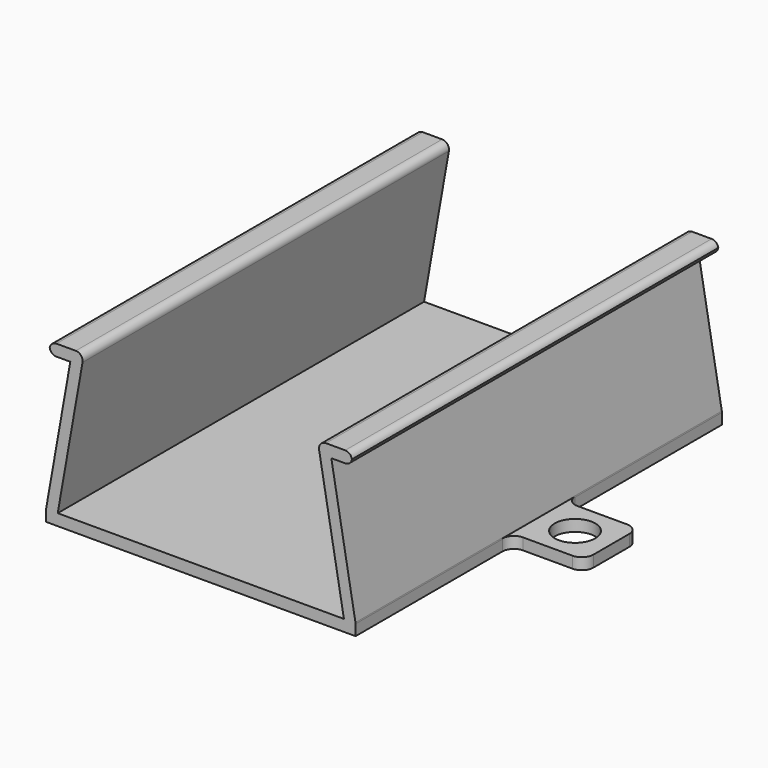
from build123d import *

# Parameters (mm, degrees)
F1_DEPTH    = 25.4
F2_T1_DEPTH = 55.3405811878
F2_T3_DEPTH = 54.61
F2_T5_DEPTH = 51.133331808
F3_R        = 2.2479
F4_DEPTH    = 1.27


# Not quite as in the source:
# - a fillet or chamfer that OpenCascade refuses, or shapes differently, is made with other operations: its cross-section is extruded or revolved along the edge and cut away or added


with BuildPart() as f1:
    # F0 (on Front) → F1 (new body, symmetric)
    with BuildSketch(Plane.XZ):
        Polygon((-14.4773686111, 15.875), (-17.1645917971, 0.635), (-15.875, 0.635), (-12.9638415485, 17.145), (-16.7738415485, 17.145), (-16.7738415485, 15.875), align=None)
        Polygon((-15.875, 0.635), (-17.1645917971, 0.635), (-17.1645917971, -0.635), (17.1645917971, -0.635), (17.1645917971, 0.635), (15.875, 0.635), align=None)
        Polygon((12.9638415485, 17.145), (15.875, 0.635), (17.1645917971, 0.635), (14.4773686111, 15.875), (16.7738415485, 15.875), (16.7738415485, 17.145), align=None)
    extrude(amount=F1_DEPTH, both=True)

    # F2: fillet of radius 0.762 on 8 edges, made by hand

    # F2_s2 → F2_t1 (cut)
    with BuildSketch(Plane.XZ.offset(-27.6702905939)):
        with BuildLine():
            ThreePointArc((-13.8719577861, 17.145), (-13.2882319204, 16.8728041586), (-13.1215342783, 16.2506800886))
            Line((-13.1215342783, 16.2506800886), (-12.9638415485, 17.145))
            Line((-12.9638415485, 17.145), (-13.8719577861, 17.145))
        make_face()
        with BuildLine():
            ThreePointArc((13.1215342783, 16.2506800886), (13.2882319204, 16.8728041586), (13.8719577861, 17.145))
            Line((13.8719577861, 17.145), (12.9638415485, 17.145))
            Line((12.9638415485, 17.145), (13.1215342783, 16.2506800886))
        make_face()
    extrude(amount=F2_T1_DEPTH, mode=Mode.SUBTRACT)

    # F2_s4 → F2_t3 (cut)
    with BuildSketch(Plane.XZ.offset(-27.305)):
        with BuildLine():
            ThreePointArc((-16.7738415485, 16.383), (-16.5506569158, 16.9218153673), (-16.0118415485, 17.145))
            Line((-16.0118415485, 17.145), (-16.7738415485, 17.145))
            Line((-16.7738415485, 17.145), (-16.7738415485, 16.383))
        make_face()
        with BuildLine():
            ThreePointArc((16.0118415485, 17.145), (16.5506569158, 16.9218153673), (16.7738415485, 16.383))
            Line((16.7738415485, 16.383), (16.7738415485, 17.145))
            Line((16.7738415485, 17.145), (16.0118415485, 17.145))
        make_face()
        with BuildLine():
            ThreePointArc((-16.0118415485, 15.875), (-16.5506569158, 16.0981846327), (-16.7738415485, 16.637))
            Line((-16.7738415485, 16.637), (-16.7738415485, 15.875))
            Line((-16.7738415485, 15.875), (-16.0118415485, 15.875))
        make_face()
        with BuildLine():
            ThreePointArc((16.7738415485, 16.637), (16.5506569158, 16.0981846327), (16.0118415485, 15.875))
            Line((16.0118415485, 15.875), (16.7738415485, 15.875))
            Line((16.7738415485, 15.875), (16.7738415485, 16.637))
        make_face()
    extrude(amount=F2_T3_DEPTH, mode=Mode.SUBTRACT)

    # F2_s6 → F2_t5 (cut)
    with BuildSketch(Plane.XZ.offset(-25.566665904)):
        with BuildLine():
            ThreePointArc((-17.1530153049, 0.7006535498), (-17.161692157, 0.6347463144), (-17.1645917971, 0.5683336384))
            Line((-17.1645917971, 0.5683336384), (-17.1645917971, 0.635))
            Line((-17.1645917971, 0.635), (-17.1530153049, 0.7006535498))
        make_face()
        with BuildLine():
            ThreePointArc((17.1530153049, 0.7006535498), (17.161692157, 0.6347463144), (17.1645917971, 0.5683336384))
            Line((17.1645917971, 0.5683336384), (17.1645917971, 0.635))
            Line((17.1645917971, 0.635), (17.1530153049, 0.7006535498))
        make_face()
    extrude(amount=F2_T5_DEPTH, mode=Mode.SUBTRACT)

    # F3 (on face) → F4 (join)
    with BuildSketch(Plane(origin=(0, 0, -0.635), x_dir=(1, 0, 0), z_dir=(0, 0, -1))):
        with BuildLine():
            Line((-17.1645917971, 3.7719), (-17.1645917971, 5.0419))
            ThreePointArc((-17.1645917971, 5.0419), (-17.536566185, 4.1438743879), (-18.4345917971, 3.7719))
            Line((-18.4345917971, 3.7719), (-23.9463917971, 3.7719))
            ThreePointArc((-23.9463917971, 3.7719), (-24.8444174092, 3.3999256121), (-25.2163917971, 2.5019))
            Line((-25.2163917971, 2.5019), (-25.2163917971, -2.5019))
            ThreePointArc((-25.2163917971, -2.5019), (-24.8444174092, -3.3999256121), (-23.9463917971, -3.7719))
            Line((-23.9463917971, -3.7719), (-18.4345917971, -3.7719))
            ThreePointArc((-18.4345917971, -3.7719), (-17.536566185, -4.1438743879), (-17.1645917971, -5.0419))
            Line((-17.1645917971, -5.0419), (-17.1645917971, -3.7719))
            Line((-17.1645917971, -3.7719), (-17.1645917971, 3.7719))
        make_face()
        with Locations((-21.1904917971, 0)):
            Circle(F3_R, mode=Mode.SUBTRACT)
        with BuildLine():
            Line((23.9463917971, 3.7719), (18.4345917971, 3.7719))
            ThreePointArc((18.4345917971, 3.7719), (17.536566185, 4.1438743879), (17.1645917971, 5.0419))
            Line((17.1645917971, 5.0419), (17.1645917971, 3.7719))
            Line((17.1645917971, 3.7719), (17.1645917971, -3.7719))
            Line((17.1645917971, -3.7719), (17.1645917971, -5.0419))
            ThreePointArc((17.1645917971, -5.0419), (17.536566185, -4.1438743879), (18.4345917971, -3.7719))
            Line((18.4345917971, -3.7719), (23.9463917971, -3.7719))
            ThreePointArc((23.9463917971, -3.7719), (24.8444174092, -3.3999256121), (25.2163917971, -2.5019))
            Line((25.2163917971, -2.5019), (25.2163917971, 2.5019))
            ThreePointArc((25.2163917971, 2.5019), (24.8444174092, 3.3999256121), (23.9463917971, 3.7719))
        make_face()
        with Locations((21.1904917971, 0)):
            Circle(F3_R, mode=Mode.SUBTRACT)
    extrude(amount=-F4_DEPTH)


solid = f1.part
